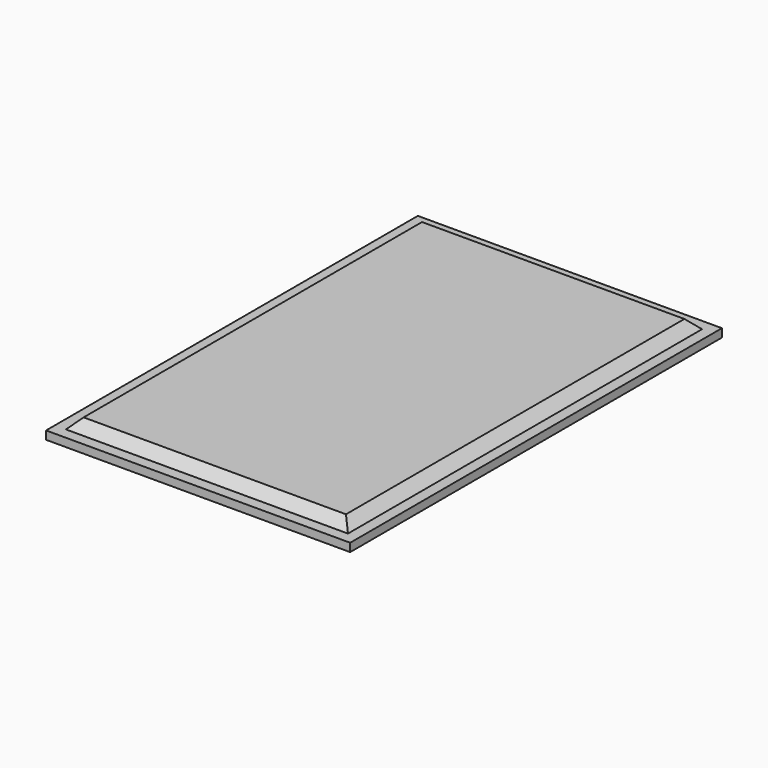
from build123d import *

# Parameters (mm, degrees)
F0_W     = 99.2
F0_H     = 151.6
F0_W_2   = 92
F0_H_2   = 144.4
F0_W_3   = 85.6
F0_H_3   = 138
F1_DEPTH = 2.7
F2_DEPTH = 3.2
F3_SIZE  = 3.19999


# Not quite as in the source:
# - a fillet or chamfer is up to 0.001 mm smaller than in the source, because OpenCascade refuses the exact size


with BuildPart() as f1:
    # F0 (on Top) → F1 (new body)
    with BuildSketch(Plane.XY):
        Rectangle(F0_W, F0_H)
        Rectangle(F0_W_2, F0_H_2, mode=Mode.SUBTRACT)
        Rectangle(F0_W_2, F0_H_2)
        Rectangle(F0_W_3, F0_H_3, mode=Mode.SUBTRACT)
        Rectangle(F0_W_3, F0_H_3)
    extrude(amount=-F1_DEPTH)

    # F0 (on Top) → F2 (join)
    with BuildSketch(Plane.XY):
        Rectangle(F0_W_2, F0_H_2)
        Rectangle(F0_W_3, F0_H_3, mode=Mode.SUBTRACT)
        Rectangle(F0_W_3, F0_H_3)
    extrude(amount=F2_DEPTH)

    # F3 (size 3.2 in the source; OpenCascade refuses exactly that, so slightly less here)
    f3_edges = [f1.edges().sort_by_distance(p)[0] for p in [
        (0, -72.2, 3.2),
        (-46, 0, 3.2),
        (46, 0, 3.2),
        (0, 72.2, 3.2),
    ]]
    chamfer(f3_edges, length=F3_SIZE)


solid = f1.part
